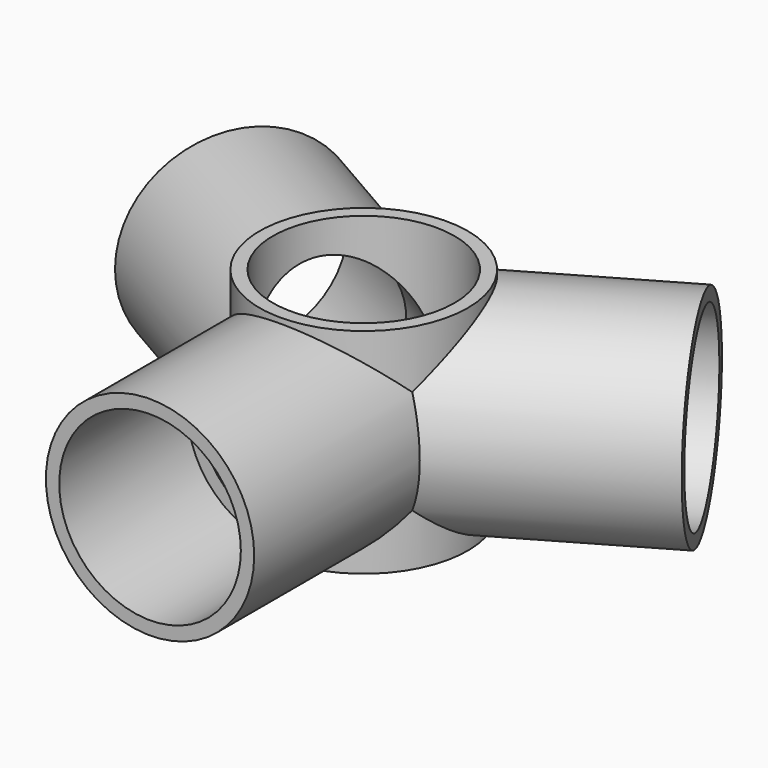
from build123d import *
from build123d import SkipClean  # not in build123d's __all__

# Parameters (mm, degrees)
F0_R             = 19.5
F0_R_2           = 14.5
F1_DEPTH         = 40
F2_R             = 17
F3_DEPTH         = 30
F5_R             = 19.5
F6_COPIES_COUNT  = 3
F8_END_RADIUS    = 17
F7_R             = 14.5
F8_REACH         = 132.9006886826
F8_COPIES_COUNT  = 3
F8_COPIES_ANGLE  = 239.9998
F9_R             = 17
F10_DEPTH        = 30
F10_COPIES_COUNT = 3


# Not quite as in the source:
# - a pattern or mirror of a feature is missing from the dataset's text; its kind, count and spacing are read off the source's solid


with BuildPart() as f1:
    # F0 (on Top) → F1 (new body)
    with BuildSketch(Plane.XY):
        Circle(F0_R)
        Circle(F0_R_2, mode=Mode.SUBTRACT)
    extrude(amount=F1_DEPTH)

    # F2 (on face) → F3 (cut)
    with BuildSketch(Plane.XY.offset(40)):
        Circle(F2_R)
    extrude(amount=-F3_DEPTH, mode=Mode.SUBTRACT)

    # F5 (on offset) → F6 (join, up to the next surface of F1)
    with BuildSketch(Plane.XZ.offset(50)):
        with Locations((0, 19.5)):
            Circle(F5_R)
    with SkipClean():  # cleaning this boolean's faces spoils the solid; the shape is the same uncleaned
        f6 = extrude(until=Until.NEXT, dir=(0, 1, 0))

    # F6_copies: F6 ×3 about axis
    f6_copies_axis = Axis((0, 0, 0), (0, 0, 1))
    for i in range(1, F6_COPIES_COUNT):
        add(f6.rotate(f6_copies_axis, i * 360 / F6_COPIES_COUNT), clean=False)

    f8_end = (Plane.XY.offset(25) * Cylinder(F8_END_RADIUS, 557.6990366969, mode=Mode.PRIVATE)).faces().sort_by_distance((-17, 0, 25))[0]
    # F7 (on offset) → F8 (cut, up to the whole of a round face its end follows)
    with BuildSketch(Plane.XZ.offset(50)):
        with Locations((0, 19.5)):
            Circle(F7_R)
    f8_long = extrude(amount=-F8_REACH, mode=Mode.PRIVATE)
    f8 = split(f8_long, bisect_by=f8_end, keep=Keep.ALL, mode=Mode.PRIVATE).solids().sort_by_distance((0, -50, 19.5))[0]
    add(f8, mode=Mode.SUBTRACT)

    # F8_copies: F8 ×3 about axis
    f8_copies_axis = Axis((0, 0, 0), (0, 0, 1))
    for i in range(1, F8_COPIES_COUNT):
        add(f8.rotate(f8_copies_axis, i * F8_COPIES_ANGLE / (F8_COPIES_COUNT - 1)), clean=False, mode=Mode.SUBTRACT)

    # F9 (on offset) → F10 (cut)
    with BuildSketch(Plane.XZ.offset(50)):
        with Locations((0, 19.5)):
            Circle(F9_R)
    f10 = extrude(amount=-F10_DEPTH, mode=Mode.SUBTRACT)

    # F10_copies: F10 ×3 about axis
    f10_copies_axis = Axis((0, 0, 0), (0, 0, 1))
    for i in range(1, F10_COPIES_COUNT):
        add(f10.rotate(f10_copies_axis, i * 360 / F10_COPIES_COUNT), clean=False, mode=Mode.SUBTRACT)


solid = f1.part
